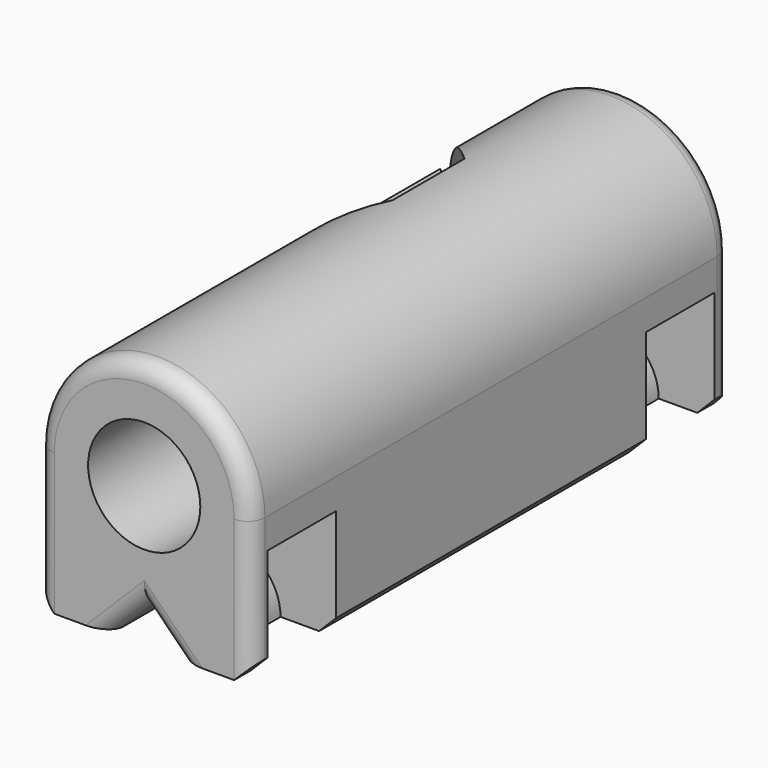
from build123d import *

# Parameters (mm, degrees)
F0_R      = 3.275
F1_DEPTH  = 17.5
F3_DEPTH  = 14.526
F5_DEPTH  = 11.1862926682
F7_DEPTH  = 35.001
F8_R      = 0.5
F9_W      = 1.5
F9_H      = 5
F12_DEPTH = 5
F13_SIZE  = 1
F14_R     = 1
F15_R     = 3.275
F16_DEPTH = 1.2


# Not quite as in the source:
# - a pattern or mirror of a feature is missing from the dataset's text; its kind, count and spacing are read off the source's solid
# - a feature names something its author has since deleted; it is built from what else it names


with BuildPart() as f1:
    # F0 (on Front) → F1 (new body, symmetric)
    with BuildSketch(Plane.XZ):
        with BuildLine():
            Line((-6.25, 8.275), (-6.25, 0))
            Line((-6.25, 0), (-2, 0))
            Line((-2, 0), (0, 2))
            Line((0, 2), (2, 0))
            Line((2, 0), (6.25, 0))
            Line((6.25, 0), (6.25, 8.275))
            ThreePointArc((6.25, 8.275), (0, 14.525), (-6.25, 8.275))
        make_face()
        with Locations((0, 8.275)):
            Circle(F0_R, mode=Mode.SUBTRACT)
    extrude(amount=F1_DEPTH, both=True)

    # F2 (on face) → F3 (cut, through all)
    with BuildSketch(Plane(origin=(0, 0, 0), x_dir=(1, 0, 0), z_dir=(0, 0, -1))):
        Polygon((-1.5, -2.5), (-6.25, 2.25), (-6.25, -12.5), (-1.5, -7.75), align=None)
    extrude(amount=-F3_DEPTH, mode=Mode.SUBTRACT)

    # F4 (on face) → F5 (join, through all)
    with BuildSketch(Plane(origin=(0, 0, 0), x_dir=(1, 0, 0), z_dir=(0, 0, -1))):
        Polygon((-4.65, 0.65), (-6.25, 2.25), (-6.25, -11.75), (-2, -7.5), (-4.65, -4.85), align=None)
    extrude(amount=-F5_DEPTH)

    # F6 (on face) → F7 (cut, through all)
    with BuildSketch(Plane.XZ.offset(17.5)):
        with BuildLine():
            Line((-6.25, 11.1862926682), (-6.25, 8.275))
            ThreePointArc((-6.25, 8.275), (-6.0674696664, 9.774437177), (-5.5305402087, 11.1862926682))
            Line((-5.5305402087, 11.1862926682), (-6.25, 11.1862926682))
        make_face()
    extrude(amount=-F7_DEPTH, mode=Mode.SUBTRACT)

    # F8
    f8_edges = [f1.edges().sort_by_distance(p)[0] for p in [
        (-2, 7.5, 5.593146),
    ]]
    fillet(f8_edges, radius=F8_R)

    # F9 (on face) → F10 (revolve, cut)
    with BuildSketch(Plane(origin=(0, 0, 0), x_dir=(1, 0, 0), z_dir=(0, 0, -1))):
        with Locations((-3.75, -13.8)):
            Rectangle(F9_W, F9_H)
    f10 = revolve(axis=Axis((0, 0.2600380681, 0), (0, -1, 0)), mode=Mode.SUBTRACT)

    # F10_copies: F10 across plane
    add(f10.mirror(Plane(origin=(0, 0, 0), x_dir=(0, 0, -1), z_dir=(0, -1, 0))), mode=Mode.SUBTRACT)

    # F11 (on face) → F12 (cut, through all)
    with BuildSketch(Plane(origin=(0, 11.3, 0), x_dir=(-1, 0, 0), z_dir=(0, 1, 0))):
        with BuildLine():
            ThreePointArc((-4.5, 0), (-3.1819805153, 3.1819805153), (0, 4.5))
            Line((0, 4.5), (-3, 4.5))
            Line((-3, 4.5), (-3, 5.2))
            Line((-3, 5.2), (-4.3, 6.5))
            Line((-4.3, 6.5), (-6.25, 6.5))
            Line((-6.25, 6.5), (-6.25, 4.5))
            Line((-6.25, 4.5), (-6.25, 0))
            Line((-6.25, 0), (-4.5, 0))
        make_face()
    f12 = extrude(amount=F12_DEPTH, mode=Mode.SUBTRACT)

    # F12_copies: F12 across plane
    add(f12.mirror(Plane(origin=(0, 0, 0), x_dir=(0, 0, -1), z_dir=(0, -1, 0))), mode=Mode.SUBTRACT)

    # F13
    f13_edges = [f1.edges().sort_by_distance(p)[0] for p in [
        (-6.25, 15, 0),
        (-6.25, -2.875, 0),
        (6.25, 0, 0),
        (6.25, -16.9, 0),
        (6.25, 16.9, 0),
    ]]
    chamfer(f13_edges, length=F13_SIZE)

    # F14
    f14_edges = [f1.edges().sort_by_distance(p)[0] for p in [
        (-1, 17.5, 1),
        (1, 17.5, 1),
        (-1, -17.5, 1),
        (1, -17.5, 1),
        (-6.25, 17.5, 4.6375),
        (0, -17.5, 14.525),
        (0, 17.5, 14.525),
        (6.25, 17.5, 4.6375),
        (-6.25, -17.5, 4.6375),
        (6.25, -17.5, 4.6375),
    ]]
    fillet(f14_edges, radius=F14_R)

    # F15 (on face) → F16 (join)
    with BuildSketch(Plane(origin=(0, 17.5, 0), x_dir=(-1, 0, 0), z_dir=(0, 1, 0))):
        with Locations((0, 8.275)):
            Circle(F15_R)
    extrude(amount=-F16_DEPTH)


solid = f1.part
